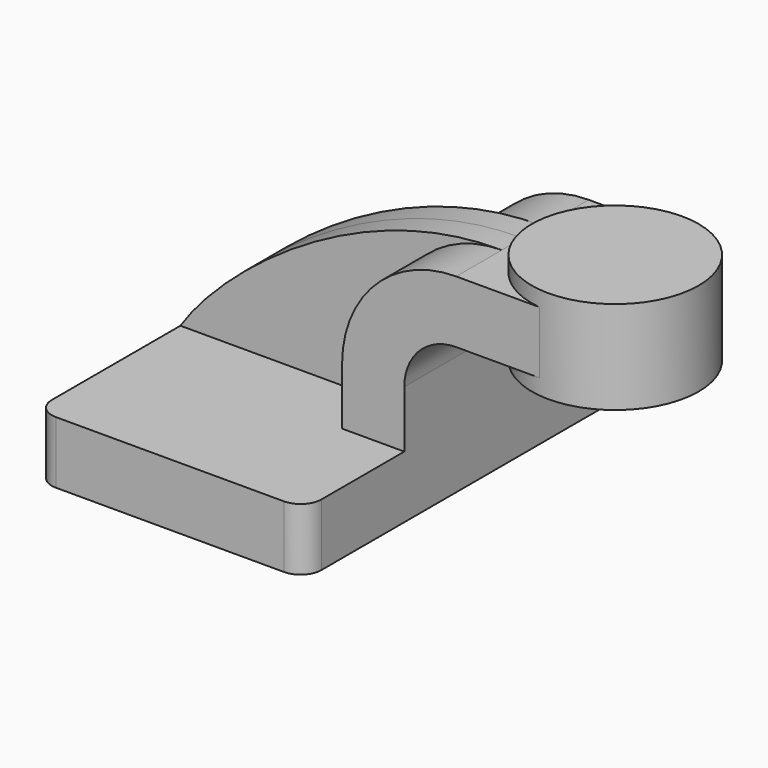
from build123d import *

# Parameters (mm, degrees)
F1_DEPTH = 63.5
F2_DEPTH = 7.9375
F3_DEPTH = 25.4
F0_W     = 25.2419677258
F0_H     = 19.05
F4_DEPTH = 25.4
F6_R     = 6.35


# Not quite as in the source:
# - a feature names something its author has since deleted; it is built from what else it names


with BuildPart() as f1:
    # F0 (on Front) → F1 (new body, symmetric)
    with BuildSketch(Plane.XZ):
        Polygon((-41.275, 9.525), (-41.275, -9.525), (41.275, -9.525), (41.275, 9.525), (22.225, 9.525), align=None)
    extrude(amount=F1_DEPTH, both=True)

    # F0 (on Front) → F2 (join, symmetric)
    with BuildSketch(Plane.XZ):
        with BuildLine():
            add(Edge.make_bspline(
                [(-41.275, 9.525), (-28.5215713084, 29.158225283), (12.6376561821, 62.4269843102), (57.15, 61.9252)],
                knots=[0, 0, 0, 0, 111.5045361635, 111.5045361635, 111.5045361635, 111.5045361635], degree=3))
            Line((-41.275, 9.525), (22.225, 9.525))
            Line((22.225, 9.525), (22.225, 27.0002))
            ThreePointArc((22.225, 27.0002), (32.4542956671, 51.6959043329), (57.15, 61.9252))
        make_face()
    extrude(amount=F2_DEPTH, both=True)

    # F0 (on Front) → F3 (join, symmetric)
    with BuildSketch(Plane.XZ):
        with BuildLine():
            Line((22.225, 9.525), (41.275, 9.525))
            Line((41.275, 9.525), (41.275, 27.0002))
            ThreePointArc((41.275, 27.0002), (45.9246798487, 38.2255201513), (57.15, 42.8752))
            Line((57.15, 42.8752), (60.325, 42.8752))
            Line((60.325, 42.8752), (60.325, 61.9252))
            Line((60.325, 61.9252), (57.15, 61.9252))
            ThreePointArc((57.15, 61.9252), (32.4542956671, 51.6959043329), (22.225, 27.0002))
            Line((22.225, 27.0002), (22.225, 9.525))
        make_face()
    extrude(amount=F3_DEPTH, both=True)

    # F0 (on Front) → F4 (join, symmetric)
    with BuildSketch(Plane.XZ):
        with Locations((72.9459838629, 52.4002)):
            Rectangle(F0_W, F0_H)
    extrude(amount=F4_DEPTH, both=True)

    # F0 (on Front) → F5 (revolve)
    with BuildSketch(Plane.XZ):
        Polygon((85.5669677258, 66.675), (85.5669677258, 61.9252), (85.5669677258, 42.8752), (85.5669677258, 38.1), (111.125, 38.1), (111.125, 66.675), align=None)
    revolve(axis=Axis((85.5669677258, 0, 52.3875), (0, 0, -1)))

    # F6
    f6_edges = [f1.edges().sort_by_distance(p)[0] for p in [
        (-41.275, -63.5, 0),
        (41.275, -63.5, 0),
        (41.275, 63.5, 0),
        (-41.275, 63.5, 0),
    ]]
    fillet(f6_edges, radius=F6_R)


solid = f1.part
